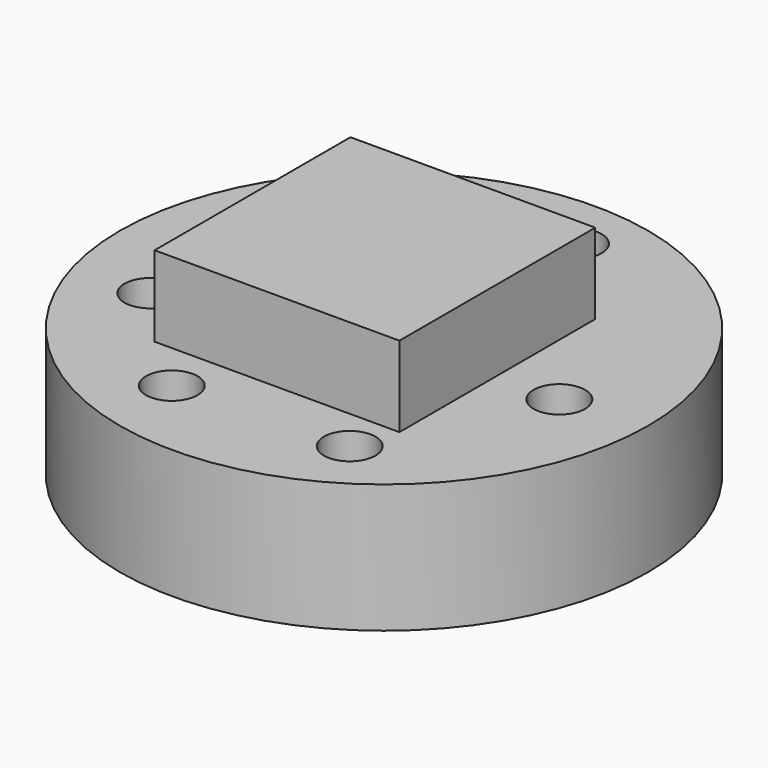
from build123d import *

# Parameters (mm, degrees)
F0_R     = 2.05
F1_DEPTH = 1
F2_W     = 1.9
F2_H     = 1.9
F3_DEPTH = 0.625
F4_R     = 0.2
F5_DEPTH = 1.001


# Not quite as in the source:
# - a feature of the source that left no trace in its solid (it failed there, or was rolled back) is left out


with BuildPart() as f1:
    # F0 (on Top) → F1 (new body)
    with BuildSketch(Plane.XY):
        Circle(F0_R)
    extrude(amount=F1_DEPTH)

    # F4 (on face) → F5 (cut, through all)
    with BuildSketch(Plane.XY.offset(1)):
        with Locations((-1.3935204645, -0.5251522966)):
            Circle(F4_R)
        with Locations((-1.4532401648, 0.5352973713)):
            Circle(F4_R)
        with Locations((1.4128740877, -0.0649337453)):
            Circle(F4_R)
        with Locations((0.8042382542, -1.3379652519)):
            Circle(F4_R)
        with Locations((-0.5337471957, -1.3917236356)):
            Circle(F4_R)
        with Locations((0.2150003766, 1.5940891608)):
            Circle(F4_R)
    extrude(amount=-F5_DEPTH, mode=Mode.SUBTRACT)


with BuildPart() as f3:
    # F2 (on face) → F3 (new body)
    with BuildSketch(Plane.XY.offset(1)):
        with Locations((-0.0252776808, -0.0563459136)):
            Rectangle(F2_W, F2_H)
    extrude(amount=F3_DEPTH)


solid = Compound([f1.part, f3.part])
